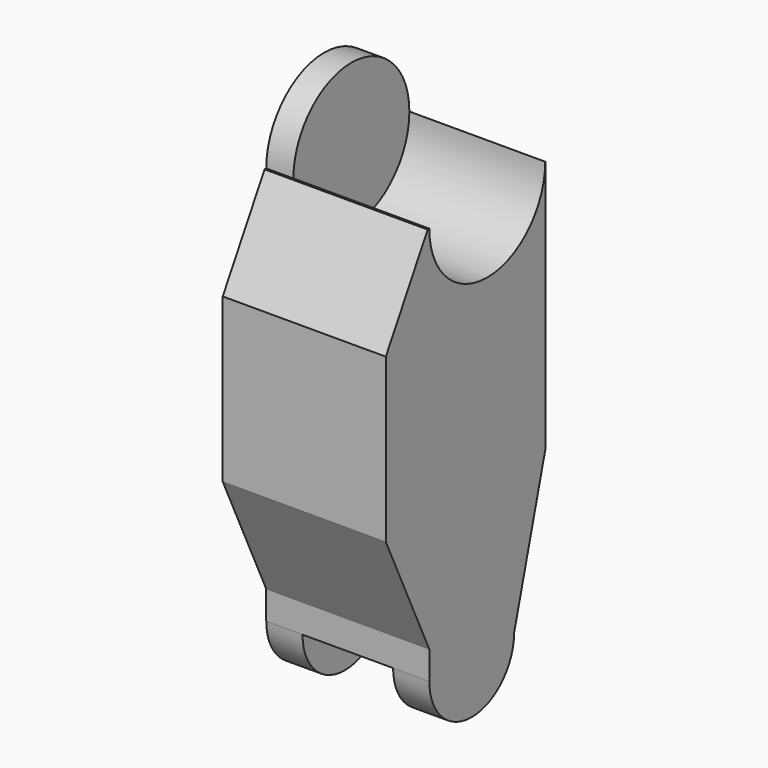
from build123d import *

# Parameters (mm, degrees)
F1_DEPTH     = 19.05
F2_DEPTH     = 114.3
F3_W         = 114.3
F3_H         = 101.6
F4_DEPTH     = 177.8
F5_T1_DEPTH  = 641.9538230647
F6_R         = 37.1475
F7_DEPTH     = 25.4
F8_R         = 37.1475
F9_DEPTH     = 25.4
F10_W        = 114.3
F10_H        = 266.7
F11_DEPTH    = 38.1
F12_T4_DEPTH = 574.9754388191
F13_T1_DEPTH = 442.85989084


# Not quite as in the source:
# - a fillet or chamfer that OpenCascade refuses, or shapes differently, is made with other operations: its cross-section is extruded or revolved along the edge and cut away or added


with BuildPart() as f1:
    # F0 (on Right) → F1 (new body)
    with BuildSketch(Plane.YZ):
        with BuildLine():
            Line((-50.8, 0), (50.8, 0))
            ThreePointArc((50.8, 0), (0, 50.8), (-50.8, 0))
        make_face()
        with BuildLine():
            Line((50.8, -101.6), (50.8, 0))
            ThreePointArc((50.8, 0), (0, -50.8), (-50.8, 0))
            Line((-50.8, 0), (-50.8, -101.6))
            Line((-50.8, -101.6), (50.8, -101.6))
        make_face()
        with BuildLine():
            ThreePointArc((-50.8, 0), (0, -50.8), (50.8, 0))
            Line((50.8, 0), (-50.8, 0))
        make_face()
    extrude(amount=F1_DEPTH)

    # F0 (on Right) → F2 (join)
    with BuildSketch(Plane.YZ):
        with BuildLine():
            Line((50.8, -101.6), (50.8, 0))
            ThreePointArc((50.8, 0), (0, -50.8), (-50.8, 0))
            Line((-50.8, 0), (-50.8, -101.6))
            Line((-50.8, -101.6), (50.8, -101.6))
        make_face()
    extrude(amount=F2_DEPTH)

    # F3 (on face) → F4 (join)
    with BuildSketch(Plane(origin=(0, 0, -101.6), x_dir=(1, 0, 0), z_dir=(0, 0, -1))):
        with Locations((57.15, 0)):
            Rectangle(F3_W, F3_H)
    extrude(amount=F4_DEPTH)

    # F5: chamfer of 101.6 x 27.223637951 on 1 edges, made by hand

    # F5_s2 → F5_t1 (cut)
    with BuildSketch(Plane.YZ.offset(-263.8269115324)):
        Polygon((23.576362049, -279.4), (50.8, -177.8), (50.8, -279.4), align=None)
    extrude(amount=F5_T1_DEPTH, mode=Mode.SUBTRACT)

    # F6 (on face) → F7 (join)
    with BuildSketch(Plane(origin=(0, 0, 0), x_dir=(0, -1, 0), z_dir=(-1, 0, 0))):
        with Locations((13.6118189755, -279.4)):
            Circle(F6_R)
    extrude(amount=-F7_DEPTH)

    # F8 (on face) → F9 (join)
    with BuildSketch(Plane.YZ.offset(114.3)):
        with Locations((-13.6118189755, -279.4)):
            Circle(F8_R)
    extrude(amount=-F9_DEPTH)

    # F10 (on face) → F11 (join)
    with BuildSketch(Plane.XZ.offset(50.8)):
        with Locations((57.15, -133.35)):
            Rectangle(F10_W, F10_H)
    extrude(amount=F11_DEPTH)

    # F12: chamfer of 88.9 x 41.45475081 on 1 edges, made by hand


with BuildPart() as f12_tool2:
    # F12_s3 → F12_t4 (new body)
    with BuildSketch(Plane.YZ.offset(-230.3377194096)):
        Polygon((-88.9, -177.8), (-47.44524919, -266.7), (-88.9, -266.7), align=None)
    extrude(amount=F12_T4_DEPTH)

    split(bisect_by=Plane.XZ.offset(50.8), keep=Keep.TOP)


with BuildPart() as f1_1:
    add(f1.part)

    # F12_t1: cut F12_tool2
    add(f12_tool2.part, mode=Mode.SUBTRACT)

    # F13: chamfer of 63.5 x 36.6617420935 on 1 edges, made by hand

    # F13_s2 → F13_t1 (cut)
    with BuildSketch(Plane.YZ.offset(-164.27994542)):
        Polygon((-88.9, -63.5), (-52.2382579065, 0), (-88.9, 0), align=None)
    extrude(amount=F13_T1_DEPTH, mode=Mode.SUBTRACT)


solid = f1_1.part
